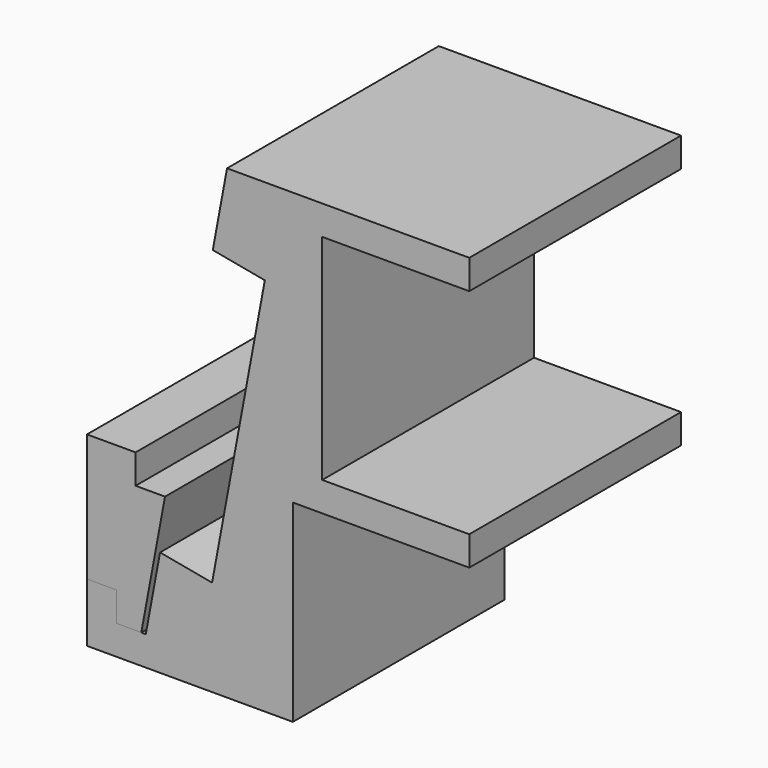
from build123d import *

# Parameters (mm, degrees)
F1_DEPTH = 90
F2_DEPTH = 90


# Not quite as in the source:
# - a feature names something its author has since deleted; it is built from what else it names


with BuildPart() as f1:
    # F0 (on Front) → F1 (new body)
    with BuildSketch(Plane.XZ):
        Polygon((-40, 92.7631145057), (-40, 0), (20, 0), (20, 10), (-30, 10), (-30, 82.7631145057), (20, 82.7631145057), (20, 92.7631145057), align=None)
        Polygon((-40, -65.6878501177), (-40, 0), (-40, 92.7631145057), (-62.3719146089, 92.7631145057), (-67.2205521113, 66.7104617738), (-49.5244106331, 63.4170476212), (-58.4898158262, 15.2442180415), (-67.4552210193, -32.9286115383), (-85.1513624976, -29.6351973858), (-90, -55.6878501177), (-91.5257563369, -55.6878501177), (-100, -55.6878501177), (-100, -45.6878501177), (-110, -45.6878501177), (-110, -65.6878501177), align=None)
    extrude(amount=F1_DEPTH)


with BuildPart() as f2:
    # F0 (on Front) → F2 (new body)
    with BuildSketch(Plane.XZ):
        Polygon((-110, -2.3839132024), (-110, -45.6878501177), (-100, -45.6878501177), (-100, -55.6878501177), (-91.5257563369, -55.6878501177), (-83.4664967026, -12.3839132024), (-93.4664967026, -12.3839132024), (-93.4664967026, -2.3839132024), align=None)
    extrude(amount=F2_DEPTH)


solid = Compound([f1.part, f2.part])
